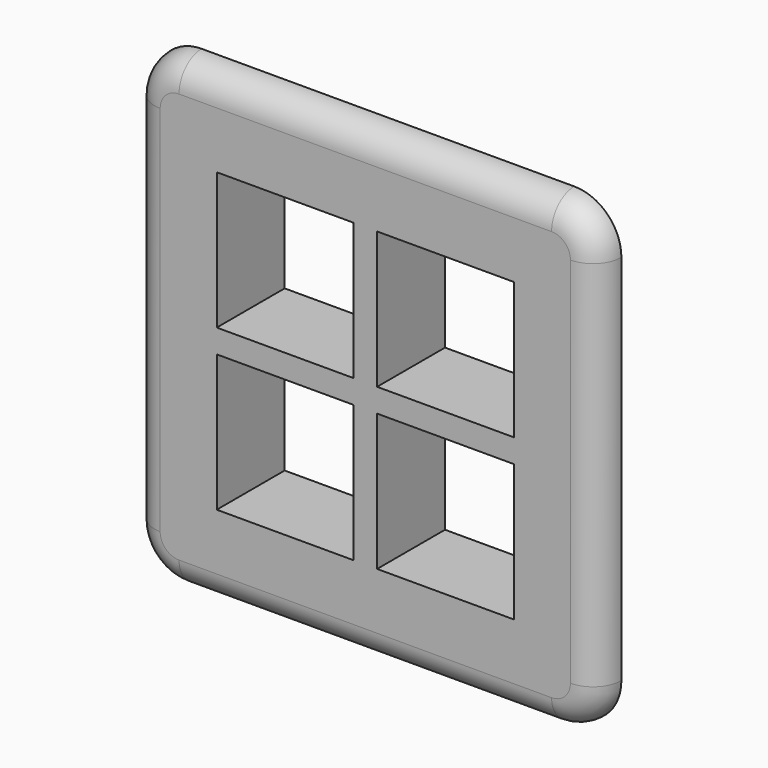
from build123d import *

# Parameters (mm, degrees)
F0_W     = 7.5
F0_H     = 7.5
F0_W_2   = 0.1
F0_H_2   = 0.1
F0_H_3   = 2.9
F0_W_3   = 0.3
F0_W_4   = 2.9
F1_DEPTH = 1.8
F2_W     = 0.6
F2_H     = 7.5
F3_DEPTH = 1.2
F4_W     = 0.6
F4_H     = 7.5
F5_DEPTH = 1.2
F7_DEPTH = 1.2
F9_DEPTH = 1.2
F10_R    = 1
F11_R    = 0.59999


# Not quite as in the source:
# - a fillet or chamfer is up to 0.001 mm smaller than in the source, because OpenCascade refuses the exact size


with BuildPart() as f1:
    # F0 (on Front) → F1 (new body)
    with BuildSketch(Plane.XZ):
        with Locations((-0.15, 3.15)):
            Rectangle(F0_W, F0_H)
        Polygon((-0.3, 3), (-0.3, 2.9), (-0.3, 0), (-0.4, 0), (-3.3, 0), (-3.3, 2.9), (-3.3, 3), (-0.4, 3), align=None, mode=Mode.SUBTRACT)
        Polygon((0.1, 0), (0, 0), (0, 2.9), (0, 3), (0.1, 3), (3, 3), (3, 2.9), (3, 0), align=None, mode=Mode.SUBTRACT)
        Polygon((0.1, 3.3), (0, 3.3), (-0.3, 3.3), (-0.4, 3.3), (-3.3, 3.3), (-3.3, 3.4), (-3.3, 6.3), (-0.4, 6.3), (-0.3, 6.3), (-0.3, 3.4), (0, 3.4), (0, 6.3), (0.1, 6.3), (3, 6.3), (3, 3.4), (3, 3.3), align=None, mode=Mode.SUBTRACT)
        with Locations((-0.35, 3.35)):
            Rectangle(F0_W_2, F0_H_2)
        with Locations((-0.35, 4.85)):
            Rectangle(F0_W_2, F0_H_3)
        with Locations((0.05, 3.35)):
            Rectangle(F0_W_2, F0_H_2)
        with Locations((0.05, 4.85)):
            Rectangle(F0_W_2, F0_H_3)
        with Locations((-0.15, 3.35)):
            Rectangle(F0_W_3, F0_H_2)
        with Locations((-1.85, 3.35)):
            Rectangle(F0_W_4, F0_H_2)
        with Locations((1.55, 3.35)):
            Rectangle(F0_W_4, F0_H_2)
        with Locations((1.55, 2.95)):
            Rectangle(F0_W_4, F0_H_2)
        with Locations((-1.85, 2.95)):
            Rectangle(F0_W_4, F0_H_2)
        with Locations((-0.35, 1.45)):
            Rectangle(F0_W_2, F0_H_3)
        with Locations((0.05, 1.45)):
            Rectangle(F0_W_2, F0_H_3)
        with Locations((0.05, 2.95)):
            Rectangle(F0_W_2, F0_H_2)
        with Locations((-0.35, 2.95)):
            Rectangle(F0_W_2, F0_H_2)
    extrude(amount=F1_DEPTH)

    # F2 (on face) → F3 (join)
    with BuildSketch(Plane(origin=(-3.9, 0, 0), x_dir=(0, -1, 0), z_dir=(-1, 0, 0))):
        with Locations((1.5, 3.15)):
            Rectangle(F2_W, F2_H)
    extrude(amount=F3_DEPTH)

    # F4 (on face) → F5 (join)
    with BuildSketch(Plane.YZ.offset(3.6)):
        with Locations((-1.5, 3.15)):
            Rectangle(F4_W, F4_H)
    extrude(amount=F5_DEPTH)

    # F6 (on face) → F7 (join)
    with BuildSketch(Plane.XY.offset(6.9)):
        Polygon((-5.1, -1.2), (-5.1, -1.2278293749), (-5.1, -1.8), (4.8, -1.8), (4.8, -1.2), (3.6, -1.2), (-3.9, -1.2), align=None)
    extrude(amount=F7_DEPTH)

    # F8 (on face) → F9 (join)
    with BuildSketch(Plane(origin=(0, 0, -0.6), x_dir=(1, 0, 0), z_dir=(0, 0, -1))):
        Polygon((3.6, 1.2), (4.8, 1.2), (4.8, 1.8), (-5.1, 1.8), (-5.1, 1.2), (-3.9, 1.2), align=None)
    extrude(amount=F9_DEPTH)

    # F10
    f10_edges = [f1.edges().sort_by_distance(p)[0] for p in [
        (-5.1, -1.5, -1.8),
        (4.8, -1.5, -1.8),
        (4.8, -1.5, 8.1),
        (-5.1, -1.5, 8.1),
    ]]
    fillet(f10_edges, radius=F10_R)

    # F11 (radius 0.6 in the source; OpenCascade refuses exactly that, so slightly less here)
    f11_edges = [f1.edges().sort_by_distance(p)[0] for p in [
        (-5.1, -1.8, 3.15),
    ]]
    fillet(f11_edges, radius=F11_R)


solid = f1.part
